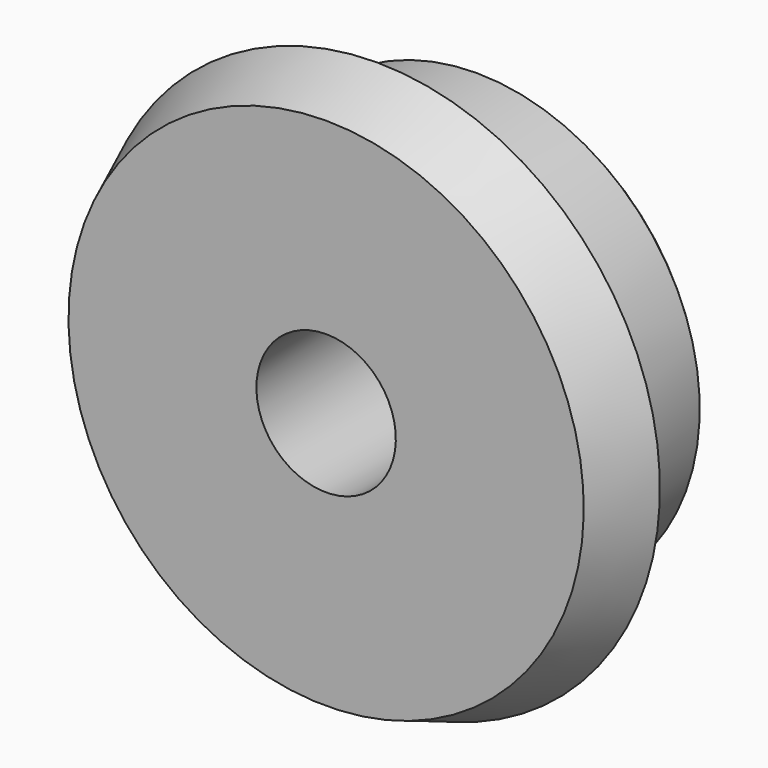
from build123d import *

# Parameters (mm, degrees)
F0_W    = 15.0114
F0_H    = 17.4625
F0_W_2  = 7.2136
F0_H_2  = 10.287
F2_R    = 1.5875
F3_SIZE = 0.79375


# Not quite as in the source:
# - a fillet or chamfer that OpenCascade refuses, or shapes differently, is made with other operations: its cross-section is extruded or revolved along the edge and cut away or added


with BuildPart() as f1:
    # F0 (on Right) → F1 (revolve)
    with BuildSketch(Plane.YZ):
        with Locations((14.7193, 16.66875)):
            Rectangle(F0_W, F0_H)
        with Locations((3.6068, 16.66875)):
            Rectangle(F0_W_2, F0_H)
        with Locations((3.6068, 30.5435)):
            Rectangle(F0_W_2, F0_H_2)
    revolve(axis=Axis((0, 25.4, 0), (0, 1, 0)))

    # F2
    f2_edges = [f1.edges().sort_by_distance(p)[0] for p in [
        (0, 7.2136, -25.4),
    ]]
    fillet(f2_edges, radius=F2_R)

    # F3
    f3_edges = [f1.edges().sort_by_distance(p)[0] for p in [
        (0, 22.225, -25.4),
    ]]
    chamfer(f3_edges, length=F3_SIZE)

    # F4: chamfer of 6.35 x 15.748 on 1 edges, made by hand

    # F4_s1 → F4_t2 (revolve, cut)
    with BuildSketch(Plane.YZ):
        Polygon((15.748, 35.687), (0, 29.337), (0, 35.687), align=None)
    revolve(axis=Axis((0, 0, 0), (0, 1, 0)), mode=Mode.SUBTRACT)


solid = f1.part
